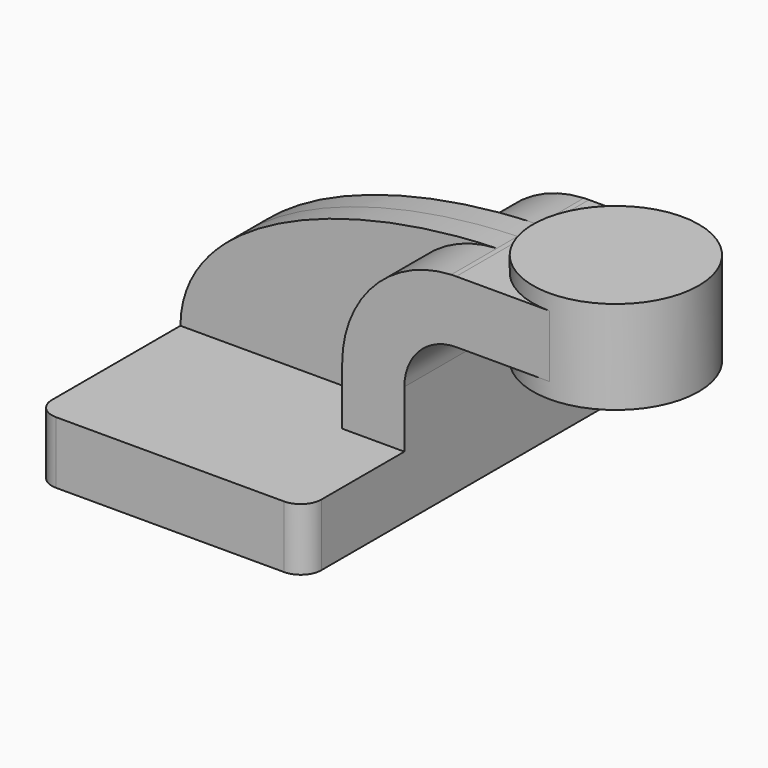
from build123d import *

# Parameters (mm, degrees)
F1_DEPTH = 63.5
F0_W     = 25.4
F0_H     = 19.05
F2_DEPTH = 25.4
F3_DEPTH = 7.9375
F5_R     = 6.35


# Not quite as in the source:
# - a feature names something its author has since deleted; it is built from what else it names


with BuildPart() as f1:
    # F0 (on Front) → F1 (new body, symmetric)
    with BuildSketch(Plane.XZ):
        Polygon((-41.275, 9.525), (-41.275, -9.525), (41.275, -9.525), (41.275, 9.525), (22.225, 9.525), align=None)
    extrude(amount=F1_DEPTH, both=True)

    # F0 (on Front) → F2 (join, symmetric)
    with BuildSketch(Plane.XZ):
        with BuildLine():
            Line((22.225, 9.525), (41.275, 9.525))
            Line((41.275, 9.525), (41.275, 27.0002))
            ThreePointArc((41.275, 27.0002), (45.9246798487, 38.2255201513), (57.15, 42.8752))
            Line((57.15, 42.8752), (60.325, 42.8752))
            Line((60.325, 42.8752), (60.325, 61.9252))
            Line((60.325, 61.9252), (57.15, 61.9252))
            add(Edge.make_bspline(
                [(55.607749268, 61.89113131), (56.1221853633, 61.9046338014), (56.6362918319, 61.9159921928), (57.15, 61.9252)],
                knots=[110.2962801392, 110.2962801392, 110.2962801392, 110.2962801392, 111.5045361635, 111.5045361635, 111.5045361635, 111.5045361635], degree=3))
            ThreePointArc((55.607749268, 61.89113131), (31.9149179532, 51.1444800491), (22.225, 27.0002))
            Line((22.225, 27.0002), (22.225, 9.525))
        make_face()
        with Locations((73.025, 52.4002)):
            Rectangle(F0_W, F0_H)
    extrude(amount=F2_DEPTH, both=True)

    # F0 (on Front) → F3 (join, symmetric)
    with BuildSketch(Plane.XZ):
        with BuildLine():
            add(Edge.make_bspline(
                [(-41.275, 9.525), (-41.060178382, 41.5590820395), (8.6471825165, 60.6585493514), (55.607749268, 61.89113131)],
                knots=[0, 0, 0, 0, 110.2962801392, 110.2962801392, 110.2962801392, 110.2962801392], degree=3))
            Line((-41.275, 9.525), (22.225, 9.525))
            Line((22.225, 9.525), (22.225, 27.0002))
            ThreePointArc((22.225, 27.0002), (31.9149179532, 51.1444800491), (55.607749268, 61.89113131))
        make_face()
    extrude(amount=F3_DEPTH, both=True)

    # F0 (on Front) → F4 (revolve)
    with BuildSketch(Plane.XZ):
        Polygon((85.725, 66.675), (85.725, 61.9252), (85.725, 42.8752), (85.725, 38.1), (111.125, 38.1), (111.125, 66.675), align=None)
    revolve(axis=Axis((85.725, 0, 52.3875), (0, 0, -1)))

    # F5
    f5_edges = [f1.edges().sort_by_distance(p)[0] for p in [
        (41.275, -63.5, 0),
        (41.275, 63.5, 0),
        (-41.275, -63.5, 0),
        (-41.275, 63.5, 0),
    ]]
    fillet(f5_edges, radius=F5_R)


solid = f1.part
